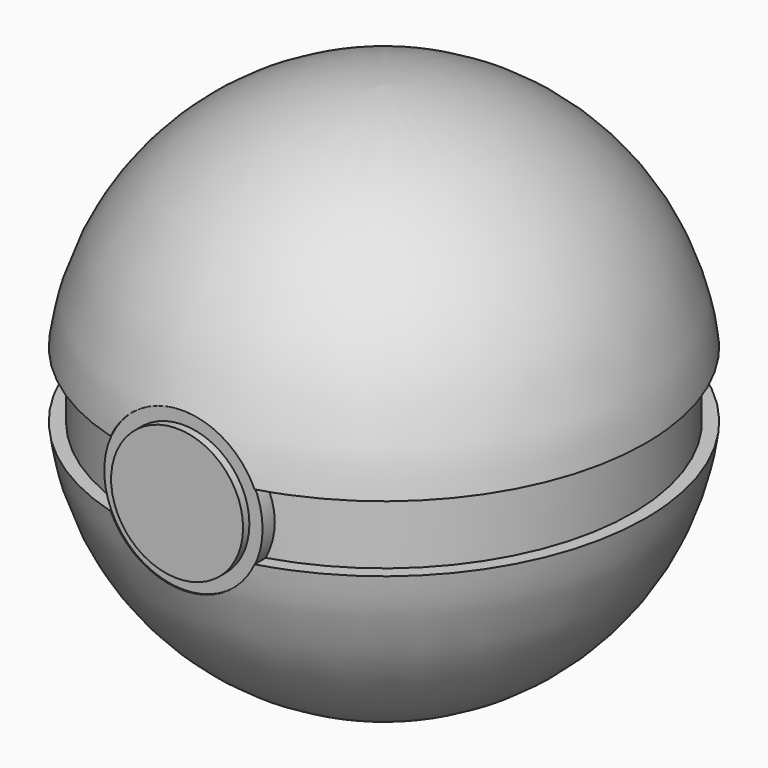
from build123d import *

# Parameters (mm, degrees)
F0_R          = 50
F1_DEPTH      = 50
F2_R          = 49.99999
F3_DEPTH      = 50
F4_R          = 49.99999
F6_R          = 15
F7_DEPTH      = 2.5
F7_DEPTH_BACK = 10
F8_W          = 11.879876256
F8_H          = 12.5124454498
F10_W         = 5.5049955845
F10_H         = 12.8705808893
F13_R         = 15
F13_R_2       = 12.5
F14_DEPTH     = 10
F15_R         = 12.5
F16_DEPTH     = 11.5


# Not quite as in the source:
# - a fillet or chamfer is up to 0.001 mm smaller than in the source, because OpenCascade refuses the exact size


with BuildPart() as f1:
    # F0 (on Top) → F1 (new body)
    with BuildSketch(Plane.XY):
        Circle(F0_R)
    extrude(amount=F1_DEPTH)

    # F2 (radius 50 in the source; OpenCascade refuses exactly that, so slightly less here)
    f2_edges = [f1.edges().sort_by_distance(p)[0] for p in [
        (-50, 0, 50),
    ]]
    fillet(f2_edges, radius=F2_R)


with BuildPart() as f3:
    # F3 (new): a face of the model
    f3_faces = [f1.part.faces().sort_by_distance(p)[0] for p in [
        (0, 0, 0),
    ]]
    extrude(f3_faces, amount=F3_DEPTH)

    # F4 (radius 50 in the source; OpenCascade refuses exactly that, so slightly less here)
    f4_edges = [f3.edges().sort_by_distance(p)[0] for p in [
        (-50, 0, -50),
    ]]
    fillet(f4_edges, radius=F4_R)


with BuildPart() as f7_tool:
    # F6 (on offset) → F7 (new body, two sides)
    with BuildSketch(Plane.XZ.offset(47.5)) as f7_sk:
        Circle(F6_R)
    extrude(amount=F7_DEPTH)
    extrude(f7_sk.sketch, amount=-F7_DEPTH_BACK)


with BuildPart() as f1_1:
    add(f1.part)

    # F7: cut by f7_tool
    add(f7_tool.part, mode=Mode.SUBTRACT)


with BuildPart() as f3_1:
    add(f3.part)

    # F7: cut by f7_tool
    add(f7_tool.part, mode=Mode.SUBTRACT)


with BuildPart() as f9_tool:
    # F8 (on Right) → F9 (revolve)
    with BuildSketch(Plane.YZ):
        with Locations((-47.7190874517, 0)):
            Rectangle(F8_W, F8_H)
    revolve(axis=Axis((0, 0, 30.5323097855), (0, 0, 1)))


with BuildPart() as f1_2:
    add(f1_1.part)

    # F9: cut by f9_tool
    add(f9_tool.part, mode=Mode.SUBTRACT)


with BuildPart() as f3_2:
    add(f3_1.part)

    # F9: cut by f9_tool
    add(f9_tool.part, mode=Mode.SUBTRACT)


with BuildPart() as f11:
    # F10 (on Right) → F11 (revolve)
    with BuildSketch(Plane.YZ):
        with Locations((44.3079993129, 0)):
            Rectangle(F10_W, F10_H)
    revolve(axis=Axis((0, 0, 32.3998779058), (0, 0, 1)))

    # F13 (on face) → F14 (join)
    with BuildSketch(Plane.XZ.offset(37.5)):
        Circle(F13_R)
        Circle(F13_R_2, mode=Mode.SUBTRACT)
    extrude(amount=F14_DEPTH)


with BuildPart() as f16:
    # F15 (on face) → F16 (new body)
    with BuildSketch(Plane.XZ.offset(37.5)):
        Circle(F15_R)
    extrude(amount=F16_DEPTH)


solid = Compound([f1_2.part, f3_2.part, f11.part, f16.part])
